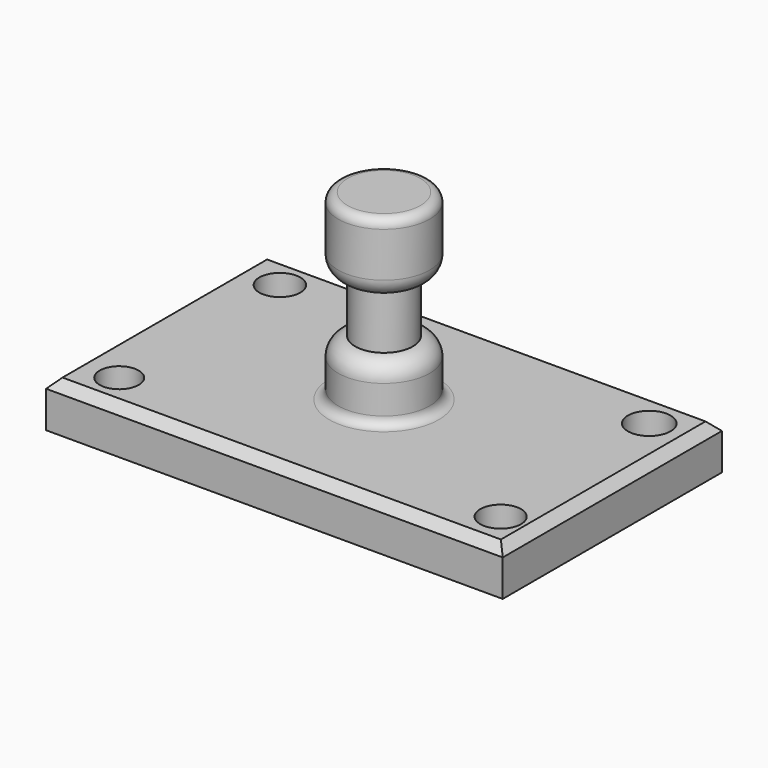
from build123d import *

# Parameters (mm, degrees)
F0_W     = 127
F0_H     = 76.2
F1_DEPTH = 12.7
F2_R     = 5.9427105428
F2_R_2   = 5.6670127921
F2_R_3   = 5.7023762048
F2_R_4   = 5.4269658504
F3_DEPTH = 12.7
F4_W     = 12.7
F4_H     = 50.8
F6_W     = 9.3170334585
F6_H     = 15.1401739568
F8_R     = 2.54
F9_SIZE  = 2.54


# Not quite as in the source:
# - a fillet or chamfer that OpenCascade refuses, or shapes differently, is made with other operations: its cross-section is extruded or revolved along the edge and cut away or added


with BuildPart() as f1:
    # F0 (on Top) → F1 (new body)
    with BuildSketch(Plane.XY):
        Rectangle(F0_W, F0_H)
    extrude(amount=F1_DEPTH)

    # F2 (on Top) → F3 (cut)
    with BuildSketch(Plane.XY):
        with Locations((52.0129092038, 27.1925590932)):
            Circle(F2_R)
        with Locations((54.2030967772, -27.1966736764)):
            Circle(F2_R_2)
        with Locations((-51.2907654047, 27.9071591794)):
            Circle(F2_R_3)
        with Locations((-51.2907616794, -27.9425289482)):
            Circle(F2_R_4)
    extrude(amount=F3_DEPTH, mode=Mode.SUBTRACT)

    # F4 (on Front) → F5 (revolve)
    with BuildSketch(Plane.XZ):
        with Locations((6.35, 38.1)):
            Rectangle(F4_W, F4_H)
    revolve(axis=Axis((0, 0, 38.1), (0, 0, 1)))

    # F6 (on Front) → F7 (revolve, cut)
    with BuildSketch(Plane.XZ):
        with Locations((12.6875618007, 35.8667755499)):
            Rectangle(F6_W, F6_H)
    revolve(axis=Axis((0, 0, 12.7), (0, 0, 1)), mode=Mode.SUBTRACT)

    # F8
    f8_edges = [f1.edges().sort_by_distance(p)[0] for p in [
        (-12.7, 0, 63.5),
        (-12.7, 0, 12.7),
    ]]
    fillet(f8_edges, radius=F8_R)

    # F9
    f9_edges = [f1.edges().sort_by_distance(p)[0] for p in [
        (0, -38.1, 12.7),
        (0, 38.1, 12.7),
        (63.5, 0, 12.7),
        (-63.5, 0, 12.7),
    ]]
    chamfer(f9_edges, length=F9_SIZE)

    # F10: fillet of radius 5.08 on 2 edges, made by hand

    # F10_s1 → F10_t2 (revolve, cut)
    with BuildSketch(Plane.XZ):
        with BuildLine():
            ThreePointArc((8.0290450715, 43.4368625283), (11.3539221311, 45.0559189466), (12.7, 48.5003674537))
            Line((12.7, 48.5003674537), (12.7, 43.4368625283))
            Line((12.7, 43.4368625283), (8.0290450715, 43.4368625283))
        make_face()
    revolve(axis=Axis((0, 0, 43.4368625283), (0, 0, 1)), mode=Mode.SUBTRACT)

    # F10_s3 → F10_t4 (revolve, cut)
    with BuildSketch(Plane.XZ):
        with BuildLine():
            ThreePointArc((12.7, 23.2331836462), (11.3539221311, 26.6776321533), (8.0290450715, 28.2966885716))
            Line((8.0290450715, 28.2966885716), (12.7, 28.2966885716))
            Line((12.7, 28.2966885716), (12.7, 23.2331836462))
        make_face()
    revolve(axis=Axis((0, 0, 28.2966885716), (0, 0, 1)), mode=Mode.SUBTRACT)


solid = f1.part
